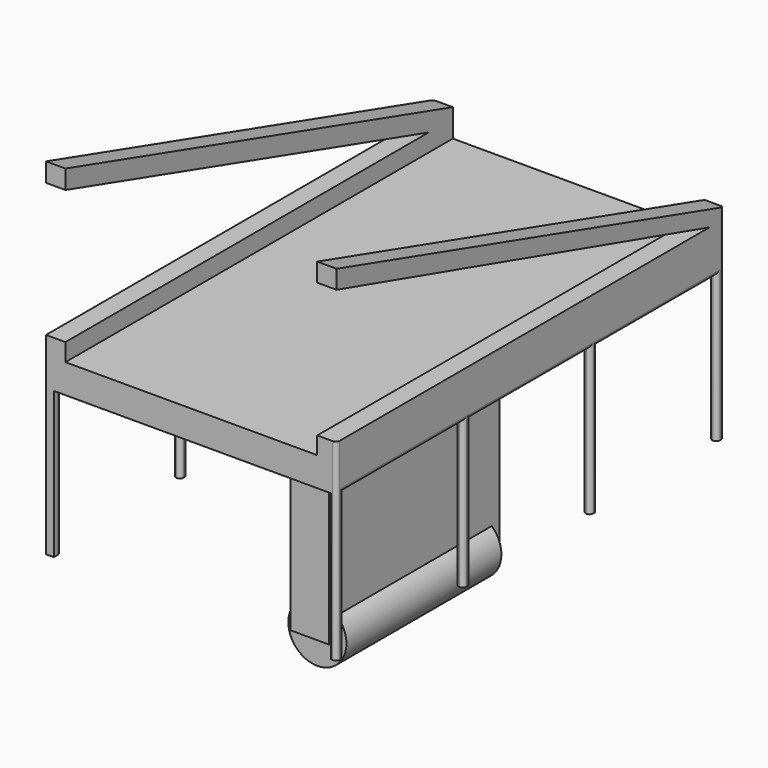
from build123d import *

# Parameters (mm, degrees)
F0_R      = 150
F1_DEPTH  = 1000
F2_W      = 200
F2_H      = 1100
F3_DEPTH  = 1200
F4_W      = 1500
F4_H      = 2500
F4_W_2    = 200
F4_H_2    = 1100
F5_DEPTH  = 150
F7_DEPTH  = 100
F9_DEPTH  = 100
F11_W     = 45
F11_H     = 755.9551119804
F11_H_2   = 734.8766446114
F11_H_3   = 716.1733627319
F11_H_4   = 701.7465054989
F12_DEPTH = 40
F13_R     = 19.99999
F14_W     = 45
F14_H     = 755.9551119804
F15_DEPTH = 40
F17_R     = 19.99999


# Not quite as in the source:
# - a fillet or chamfer is up to 0.001 mm smaller than in the source, because OpenCascade refuses the exact size


with BuildPart() as f1:
    # F0 (on Front) → F1 (new body)
    with BuildSketch(Plane.XZ):
        Circle(F0_R)
    extrude(amount=F1_DEPTH)

    # F2 (on Top) → F3 (join)
    with BuildSketch(Plane.XY):
        with Locations((0, -500)):
            Rectangle(F2_W, F2_H)
    extrude(amount=F3_DEPTH)

    # F4 (on face) → F5 (join)
    with BuildSketch(Plane.XY.offset(1200)):
        with Locations((0, -563.5802745819)):
            Rectangle(F4_W, F4_H)
        with Locations((0, -500)):
            Rectangle(F4_W_2, F4_H_2, mode=Mode.SUBTRACT)
        with Locations((0, -500)):
            Rectangle(F4_W_2, F4_H_2)
    extrude(amount=F5_DEPTH)

    # F6 (on face) → F7 (join)
    with BuildSketch(Plane.YZ.offset(750)):
        Polygon((-1813.5802745819, 1350), (686.4197254181, 1350), (686.4197254181, 1494.1539764404), (-1813.5802745819, 2229.8667430878), (-1813.5802745819, 2134.2372894287), (593.697309494, 1439.7211074829), (-1813.5802745819, 1439.7211074829), align=None)
    extrude(amount=-F7_DEPTH)


with BuildPart() as f9:
    # F8 (on face) → F9 (new body)
    with BuildSketch(Plane(origin=(-750, 0, 0), x_dir=(0, -1, 0), z_dir=(-1, 0, 0))):
        Polygon((-686.4197254181, 1350), (1813.5802745819, 1350), (1813.5802745819, 1441.313624382), (-530.3064584732, 1441.313624382), (1813.5802745819, 2132.4443817139), (1813.5802745819, 2230.1487922668), (-686.4197254181, 1492.9856567951), align=None)
    extrude(amount=-F9_DEPTH)


with BuildPart() as f1_1:
    add(f1.part)

    # F10: union F9
    add(f9.part)

    # F11 (on face) → F12 (join)
    with BuildSketch(Plane(origin=(-750, 0, 0), x_dir=(0, -1, 0), z_dir=(-1, 0, 0))):
        with Locations((1791.0802745819, 822.0224440098)):
            Rectangle(F11_W, F11_H)
        with Locations((973.0802745819, 832.5616776943)):
            Rectangle(F11_W, F11_H_2)
        with Locations((154.0802745819, 841.913318634)):
            Rectangle(F11_W, F11_H_3)
        with Locations((-663.9197254181, 849.1267472506)):
            Rectangle(F11_W, F11_H_4)
    extrude(amount=-F12_DEPTH)

    # F13 (radius 20 in the source; OpenCascade refuses exactly that, so slightly less here)
    f13_edges = [f1_1.edges().sort_by_distance(p)[0] for p in [
        (-750, -1768.580275, 822.022444),
        (-710, -1768.580275, 822.022444),
        (-750, -950.580275, 832.561678),
        (-710, -950.580275, 832.561678),
        (-750, -995.580275, 832.561678),
        (-710, -995.580275, 832.561678),
        (-750, -131.580275, 841.913319),
        (-750, -176.580275, 841.913319),
        (-710, -131.580275, 841.913319),
        (-750, 686.419725, 995.619576),
        (-750, 641.419725, 849.126747),
        (-710, 686.419725, 849.126747),
        (-710, -176.580275, 841.913319),
        (-710, 641.419725, 849.126747),
        (-750, -1382.080275, 1200),
        (-750, -563.580275, 1200),
        (-750, 254.919725, 1200),
    ]]
    fillet(f13_edges, radius=F13_R)


with BuildPart() as f15:
    # F14 (on face) → F15 (new body)
    with BuildSketch(Plane.YZ.offset(750)):
        with Locations((-1791.0802745819, 822.0224440098)):
            Rectangle(F14_W, F14_H)
    extrude(amount=-F15_DEPTH)


with BuildPart() as f15b:
    # F14 (on face) → F15, piece 2 (new body)
    with BuildSketch(Plane.YZ.offset(750)):
        with Locations((-973.0802745819, 822.0224440098)):
            Rectangle(F14_W, F14_H)
    extrude(amount=-F15_DEPTH)


with BuildPart() as f15c:
    # F14 (on face) → F15, piece 3 (new body)
    with BuildSketch(Plane.YZ.offset(750)):
        with Locations((-154.0802745819, 822.0224440098)):
            Rectangle(F14_W, F14_H)
    extrude(amount=-F15_DEPTH)


with BuildPart() as f15d:
    # F14 (on face) → F15, piece 4 (new body)
    with BuildSketch(Plane.YZ.offset(750)):
        with Locations((663.9197254181, 822.0224440098)):
            Rectangle(F14_W, F14_H)
    extrude(amount=-F15_DEPTH)


with BuildPart() as f1_2:
    add(f1_1.part)

    # F16: union F15, F15b, F15c, F15d
    add(f15.part)
    add(f15b.part)
    add(f15c.part)
    add(f15d.part)

    # F17 (radius 20 in the source; OpenCascade refuses exactly that, so slightly less here)
    f17_edges = [f1_2.edges().sort_by_distance(p)[0] for p in [
        (750, 686.419725, 969.099432),
        (710, 686.419725, 822.022444),
        (750, 641.419725, 822.022444),
        (750, -131.580275, 822.022444),
        (710, -131.580275, 822.022444),
        (750, -176.580275, 822.022444),
        (750, -950.580275, 822.022444),
        (710, -950.580275, 822.022444),
        (750, -995.580275, 822.022444),
        (710, -1768.580275, 822.022444),
        (750, -1768.580275, 822.022444),
        (750, -1813.580275, 941.882998),
        (710, -995.580275, 822.022444),
        (710, -1813.580275, 822.022444),
        (710, -176.580275, 822.022444),
        (710, 641.419725, 822.022444),
        (750, 254.919725, 1200),
        (750, -563.580275, 1200),
        (750, -1382.080275, 1200),
        (-9.999995, 686.419725, 1200),
    ]]
    fillet(f17_edges, radius=F17_R)


solid = f1_2.part
